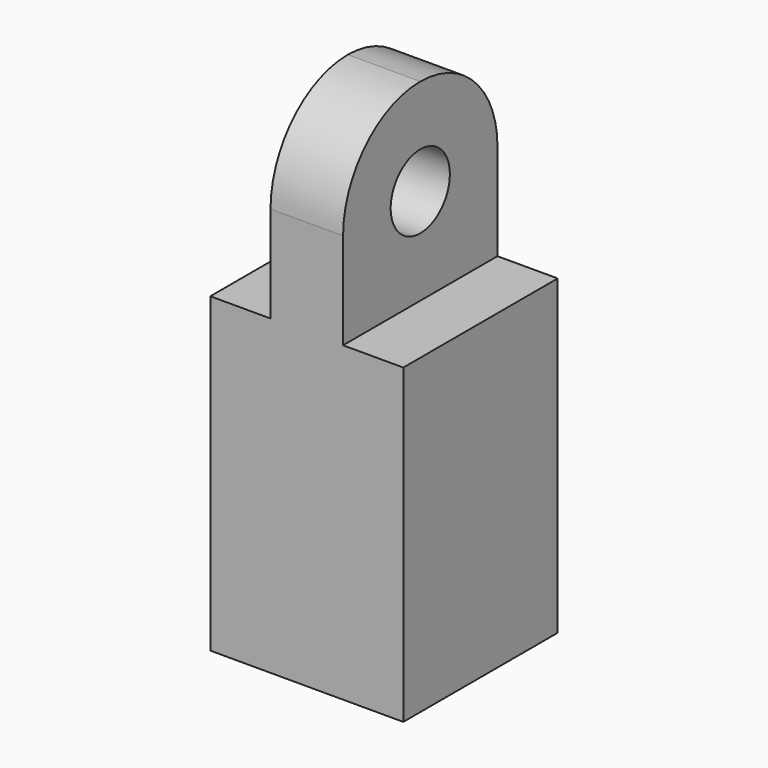
from build123d import *

# Parameters (mm, degrees)
F0_W          = 13.3
F0_H          = 13.3
F0_W_2        = 10.3
F0_H_2        = 10.3
F1_DEPTH      = 20
F2_DEPTH      = 1.5
F3_W          = 5
F3_H          = 13.3
F4_DEPTH      = 13.3
F5_T1_DEPTH   = 38.3
F6_R          = 2.55
F7_DEPTH      = 25
F7_DEPTH_BACK = 25


# Not quite as in the source:
# - a fillet or chamfer that OpenCascade refuses, or shapes differently, is made with other operations: its cross-section is extruded or revolved along the edge and cut away or added


with BuildPart() as f1:
    # F0 (on Top) → F1 (new body)
    with BuildSketch(Plane.XY):
        Rectangle(F0_W, F0_H)
        Rectangle(F0_W_2, F0_H_2, mode=Mode.SUBTRACT)
    extrude(amount=-F1_DEPTH)

    # F0 (on Top) → F2 (join)
    with BuildSketch(Plane.XY):
        Rectangle(F0_W, F0_H)
        Rectangle(F0_W_2, F0_H_2, mode=Mode.SUBTRACT)
        Rectangle(F0_W_2, F0_H_2)
    extrude(amount=F2_DEPTH)

    # F3 (on face) → F4 (join)
    with BuildSketch(Plane.XY.offset(1.5)):
        Rectangle(F3_W, F3_H)
    extrude(amount=F4_DEPTH)

    # F5: fillet of radius 6.66 on 2 edges, made by hand

    # F5_s2 → F5_t1 (cut)
    with BuildSketch(Plane.YZ.offset(-19.15)):
        with BuildLine():
            ThreePointArc((-6.65, 8.14), (-4.6993311627, 12.8493311627), (0.01, 14.8))
            Line((0.01, 14.8), (-6.65, 14.8))
            Line((-6.65, 14.8), (-6.65, 8.14))
        make_face()
        with BuildLine():
            ThreePointArc((6.65, 8.14), (4.6993311627, 12.8493311627), (-0.01, 14.8))
            Line((-0.01, 14.8), (6.65, 14.8))
            Line((6.65, 14.8), (6.65, 8.14))
        make_face()
    extrude(amount=F5_T1_DEPTH, mode=Mode.SUBTRACT)

    # F6 (on face) → F7 (cut, two sides)
    with BuildSketch(Plane.YZ.offset(2.5)) as f7_sk:
        with Locations((0, 8.14)):
            Circle(F6_R)
    extrude(amount=-F7_DEPTH, mode=Mode.SUBTRACT)
    extrude(f7_sk.sketch, amount=F7_DEPTH_BACK, mode=Mode.SUBTRACT)


solid = f1.part
